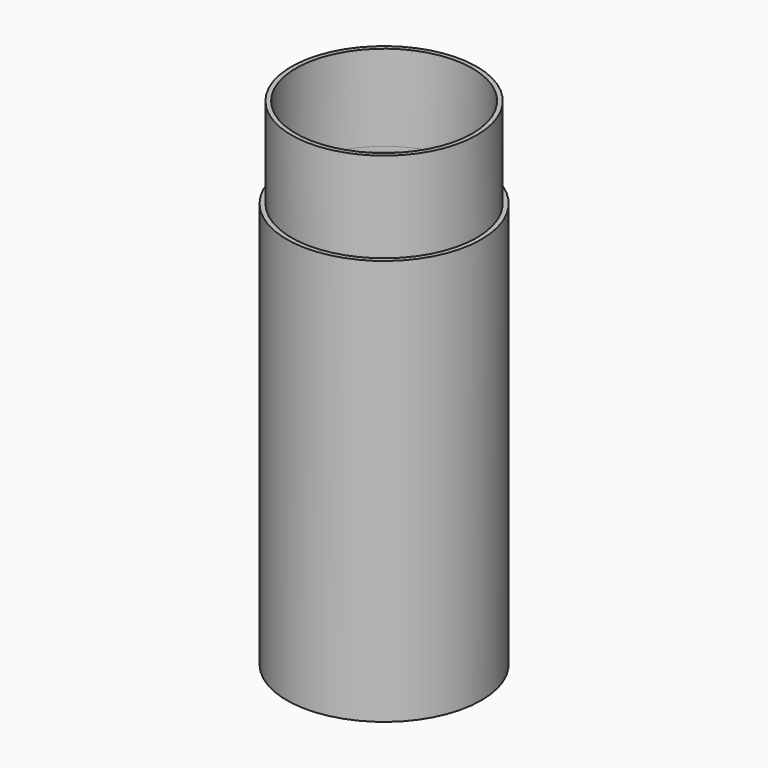
from build123d import *

# Parameters (mm, degrees)
F0_R     = 53.0991394176
F1_DEPTH = 51.71754
F0_R_2   = 55.7255834594
F2_DEPTH = 232.41034
F3_T     = -2.54
F4_DEPTH = 228.21454
F5_T     = -2.54


# Not quite as in the source:
# - a shell that OpenCascade refuses in one call is made with other operations: the cavity is built on its own and cut out


with BuildPart() as f1:
    # F0 (on Top) → F1 (new body)
    with BuildSketch(Plane.XY):
        Circle(F0_R)
    extrude(amount=F1_DEPTH)

    # F3
    f3_openings = [f1.faces().sort_by_distance(p)[0] for p in [
        (0, 0, 51.71754),
    ]]
    offset(amount=F3_T, openings=f3_openings)

    # F4 (add): a face of the model
    f4_faces = [f1.faces().sort_by_distance(p)[0] for p in [
        (0, 0, 0),
    ]]


with BuildPart() as f2:
    # F0 (on Top) → F2 (new body)
    with BuildSketch(Plane.XY):
        Circle(F0_R_2)
        Circle(F0_R, mode=Mode.SUBTRACT)
    extrude(amount=-F2_DEPTH)


with BuildPart() as f1_1:
    add(f1.part)

    add(f2.part)  # F4 merges F2
    extrude(f4_faces, amount=F4_DEPTH)

    # F5: a shell. OpenCascade refuses it in one call, so the cavity is built on its own and cut out:
    # the body offset inwards by the wall thickness, plus a prism from it out through each open face.
    f5_core = offset(f1_1.part, amount=F5_T, kind=Kind.INTERSECTION, mode=Mode.PRIVATE)
    f5_exits = [f5_core.faces().sort_by_distance(p)[0] for p in [
        (0, 0, 0),
    ]]
    add(f5_core, mode=Mode.SUBTRACT)
    extrude(f5_exits, amount=-F5_T, mode=Mode.SUBTRACT)


solid = f1_1.part
